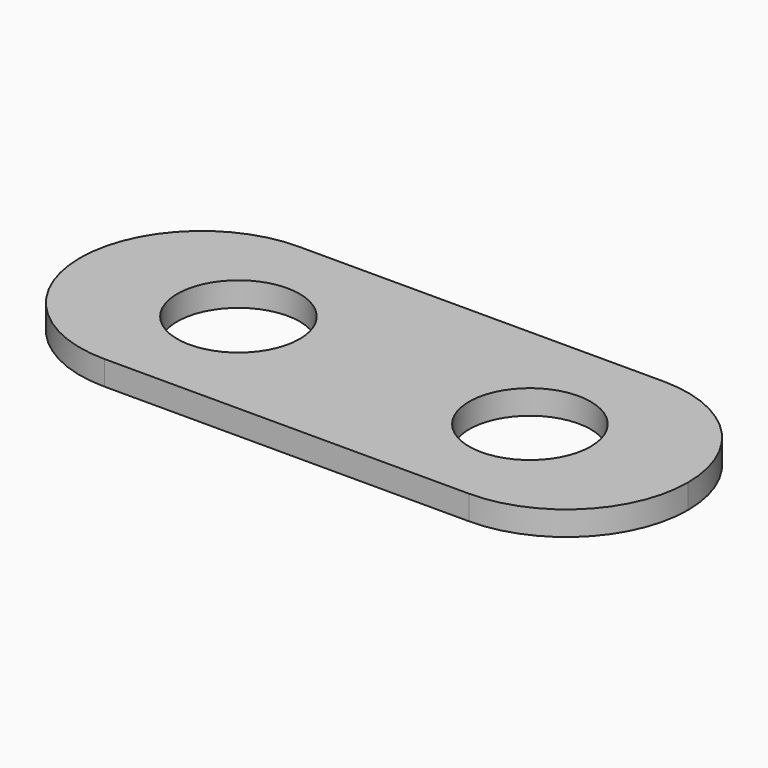
from build123d import *

# Parameters (mm, degrees)
F0_W     = 25
F0_H     = 10
F0_R     = 2.515
F0_R_2   = 2.5
F1_DEPTH = 1
F2_R     = 4.99999


# Not quite as in the source:
# - a fillet or chamfer is up to 0.001 mm smaller than in the source, because OpenCascade refuses the exact size


with BuildPart() as f1:
    # F0 (on Top) → F1 (new body)
    with BuildSketch(Plane.XY):
        Rectangle(F0_W, F0_H)
        with Locations((-5.985, 0)):
            Circle(F0_R, mode=Mode.SUBTRACT)
        with Locations((6, 0)):
            Circle(F0_R_2, mode=Mode.SUBTRACT)
    extrude(amount=F1_DEPTH)

    # F2 (radius 5 in the source; OpenCascade refuses exactly that, so slightly less here)
    f2_edges = [f1.edges().sort_by_distance(p)[0] for p in [
        (-12.5, 5, 0.5),
        (12.5, 5, 0.5),
        (12.5, -5, 0.5),
        (-12.5, -5, 0.5),
    ]]
    fillet(f2_edges, radius=F2_R)


solid = f1.part
